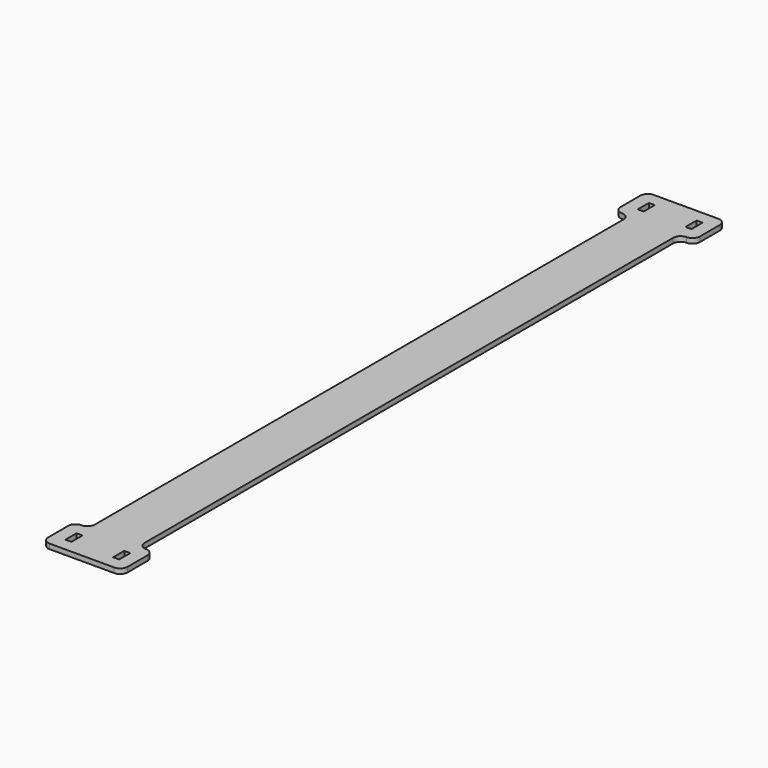
from build123d import *

# Parameters (mm, degrees)
F0_W     = 1.905
F0_H     = 4.445
F1_DEPTH = 1.5875
F2_R     = 2.38124


# Not quite as in the source:
# - a fillet or chamfer is up to 0.001 mm smaller than in the source, because OpenCascade refuses the exact size


with BuildPart() as f1:
    # F0 (on Top) → F1 (new body)
    with BuildSketch(Plane.XY):
        Polygon((-69.85, 120.65), (-95.25, 120.65), (-95.25, 107.95), (-90.4875, 107.95), (-90.4875, -107.95), (-95.25, -107.95), (-95.25, -120.65), (-69.85, -120.65), (-69.85, -107.95), (-74.6125, -107.95), (-74.6125, 107.95), (-69.85, 107.95), align=None)
        with Locations((-90.17, -114.3)):
            Rectangle(F0_W, F0_H, mode=Mode.SUBTRACT)
        with Locations((-74.93, -114.3)):
            Rectangle(F0_W, F0_H, mode=Mode.SUBTRACT)
        with Locations((-90.17, 114.3)):
            Rectangle(F0_W, F0_H, mode=Mode.SUBTRACT)
        with Locations((-74.93, 114.3)):
            Rectangle(F0_W, F0_H, mode=Mode.SUBTRACT)
    extrude(amount=F1_DEPTH)

    # F2 (radius 2.38125 in the source; OpenCascade refuses exactly that, so slightly less here)
    f2_edges = [f1.edges().sort_by_distance(p)[0] for p in [
        (-90.4875, -107.95, 0.79375),
        (-95.25, -107.95, 0.79375),
        (-95.25, -120.65, 0.79375),
        (-69.85, -120.65, 0.79375),
        (-69.85, -107.95, 0.79375),
        (-74.6125, -107.95, 0.79375),
        (-69.85, 120.65, 0.79375),
        (-69.85, 107.95, 0.79375),
        (-95.25, 120.65, 0.79375),
        (-95.25, 107.95, 0.79375),
        (-74.6125, 107.95, 0.79375),
        (-90.4875, 107.95, 0.79375),
    ]]
    fillet(f2_edges, radius=F2_R)


solid = f1.part
